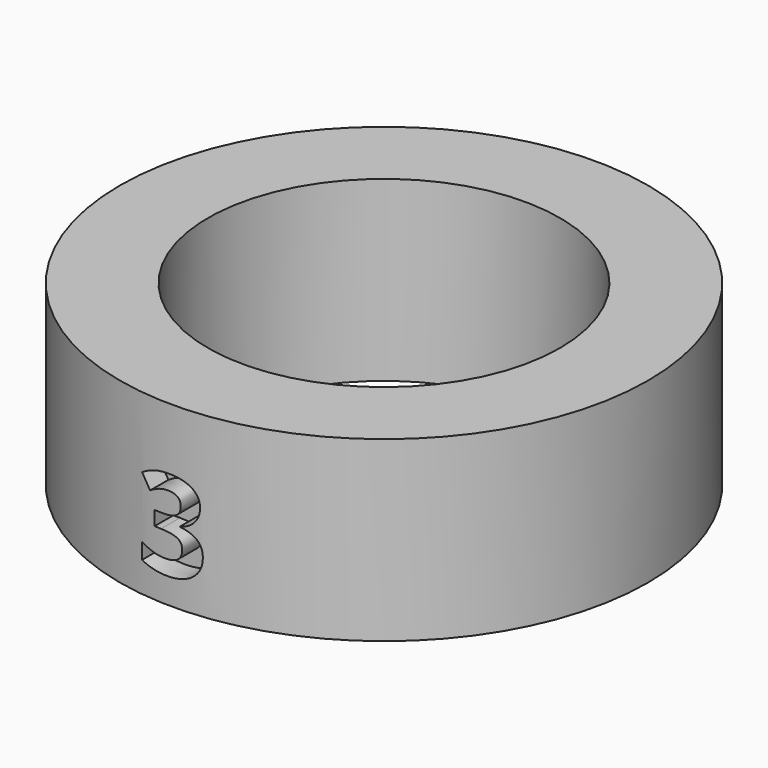
from build123d import *

# Parameters (mm, degrees)
F0_R         = 14.85
F0_R_2       = 9.9
F1_DEPTH     = 10
F3_TEXT_SIZE = 6.9444444444
F4_DEPTH     = 1.5


# Not quite as in the source:
# - Text() gives the source's letters only with a copy of the font that has no kerning and outlines rounded to 1/6400 em; it was checked with that copy


with BuildPart() as f1:
    # F0 (on Top) → F1 (new body)
    with BuildSketch(Plane.XY):
        Circle(F0_R)
        Circle(F0_R_2, mode=Mode.SUBTRACT)
    extrude(amount=F1_DEPTH)

    # F3 (on offset) → F4 (cut)
    with BuildSketch(Plane.XZ.offset(15)):
        with Locations((-2.0730251736, 1.500000013)):
            Text('3', F3_TEXT_SIZE, font='Open Sans', font_style=FontStyle.BOLD, text_align=(TextAlign.LEFT, TextAlign.BOTTOM))
    extrude(amount=-F4_DEPTH, mode=Mode.SUBTRACT)


solid = f1.part
